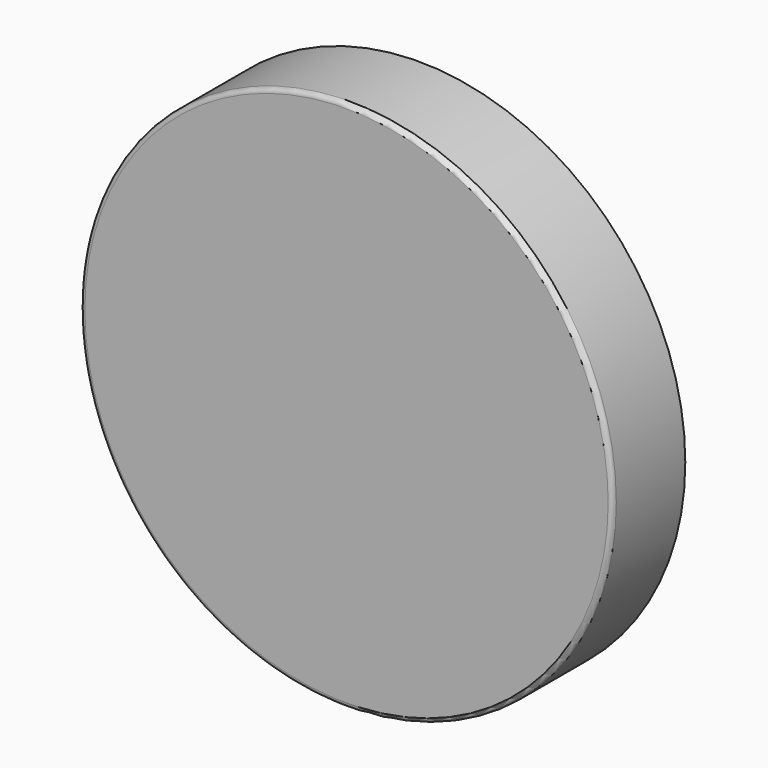
from build123d import *

# Parameters (mm, degrees)
F0_R     = 88
F1_DEPTH = 30
F2_R     = 84
F3_DEPTH = 23
F4_R     = 1.5


# Not quite as in the source:
# - a feature names something its author has since deleted; it is built from what else it names


with BuildPart() as f1:
    # F0 (on Front) → F1 (new body)
    with BuildSketch(Plane.XZ):
        Circle(F0_R)
    extrude(amount=F1_DEPTH)

    # F2 (on face) → F3 (cut)
    with BuildSketch(Plane(origin=(0, 0, 0), x_dir=(-1, 0, 0), z_dir=(0, 1, 0))):
        Circle(F2_R)
    extrude(amount=-F3_DEPTH, mode=Mode.SUBTRACT)

    # F4
    f4_edges = [f1.edges().sort_by_distance(p)[0] for p in [
        (-88, -30, 0),
    ]]
    fillet(f4_edges, radius=F4_R)


solid = f1.part
